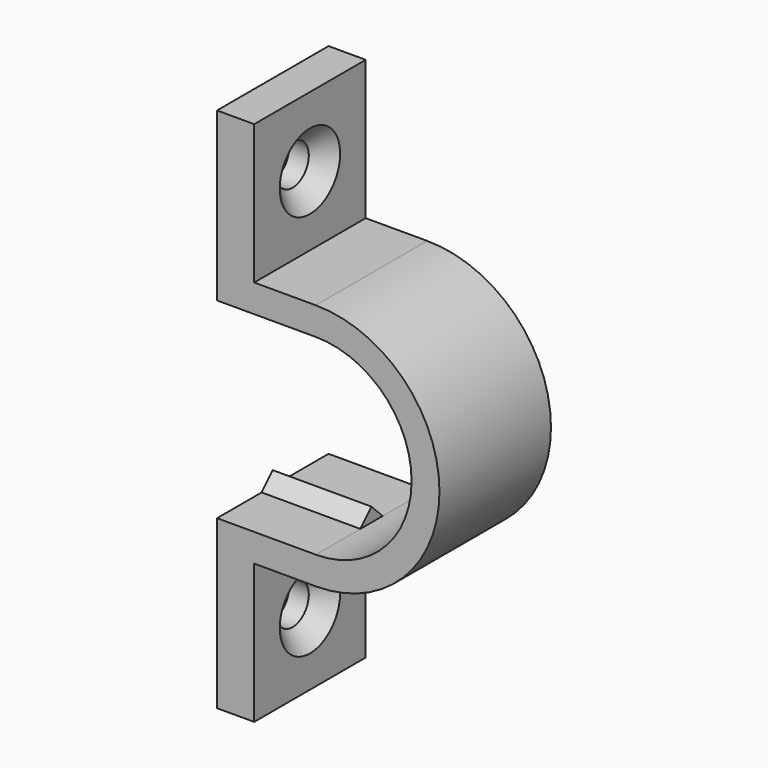
from build123d import *

# Parameters (mm, degrees)
F1_DEPTH = 12
F2_R     = 1.75
F3_DEPTH = 19.151
F4_SIZE  = 1.5
F5_W     = 8.5
F5_H     = 2.4
F6_DEPTH = 1.2
F7_W     = 8.5
F7_H     = 2.4
F8_DEPTH = 1.2
F9_SIZE  = 1.19999


# Not quite as in the source:
# - a fillet or chamfer is up to 0.001 mm smaller than in the source, because OpenCascade refuses the exact size


with BuildPart() as f1:
    # F0 (on Front) → F1 (new body)
    with BuildSketch(Plane.XZ):
        with BuildLine():
            Line((-35.8277369916, 41.9945976296), (-39.0277369916, 41.9945976296))
            Line((-39.0277369916, 41.9945976296), (-39.0277369916, 27.5945976296))
            Line((-39.0277369916, 27.5945976296), (-30.5277369916, 27.5945976296))
            ThreePointArc((-30.5277369916, 27.5945976296), (-22.2777369916, 19.3445976296), (-30.5277369916, 11.0945976296))
            Line((-30.5277369916, 11.0945976296), (-39.0277369916, 11.0945976296))
            Line((-39.0277369916, 11.0945976296), (-39.0277369916, -3.3054023704))
            Line((-39.0277369916, -3.3054023704), (-35.8277369916, -3.3054023704))
            Line((-35.8277369916, -3.3054023704), (-35.8277369916, 8.6945976296))
            Line((-35.8277369916, 8.6945976296), (-30.5277369916, 8.6945976296))
            ThreePointArc((-30.5277369916, 8.6945976296), (-19.8777369916, 19.3445976296), (-30.5277369916, 29.9945976296))
            Line((-30.5277369916, 29.9945976296), (-35.8277369916, 29.9945976296))
            Line((-35.8277369916, 29.9945976296), (-35.8277369916, 41.9945976296))
        make_face()
    extrude(amount=F1_DEPTH)

    # F2 (on face) → F3 (cut, through all)
    with BuildSketch(Plane(origin=(-39.0277369916, 0, 0), x_dir=(0, -1, 0), z_dir=(-1, 0, 0))):
        with Locations((6, 35.9945976296)):
            Circle(F2_R)
        with Locations((6, 2.6945976296)):
            Circle(F2_R)
    extrude(amount=-F3_DEPTH, mode=Mode.SUBTRACT)

    # F4
    f4_edges = [f1.edges().sort_by_distance(p)[0] for p in [
        (-35.827737, -4.25, 35.994598),
        (-35.827737, -4.25, 2.694598),
    ]]
    chamfer(f4_edges, length=F4_SIZE)

    # F5 (on face) → F6 (join)
    with BuildSketch(Plane.XY.offset(11.0945976296)):
        with Locations((-34.7777369916, -6)):
            Rectangle(F5_W, F5_H)
    extrude(amount=F6_DEPTH)

    # F7 (on face) → F8 (join)
    with BuildSketch(Plane(origin=(0, 0, 27.5945976296), x_dir=(1, 0, 0), z_dir=(0, 0, -1))):
        with Locations((-34.7777369916, 6)):
            Rectangle(F7_W, F7_H)
    extrude(amount=F8_DEPTH)

    # F9 (size 1.2 in the source; OpenCascade refuses exactly that, so slightly less here)
    f9_edges = [f1.edges().sort_by_distance(p)[0] for p in [
        (-34.777737, -7.2, 12.294598),
        (-34.777737, -4.8, 12.294598),
        (-34.777737, -7.2, 26.394598),
        (-34.777737, -4.8, 26.394598),
    ]]
    chamfer(f9_edges, length=F9_SIZE)


solid = f1.part
